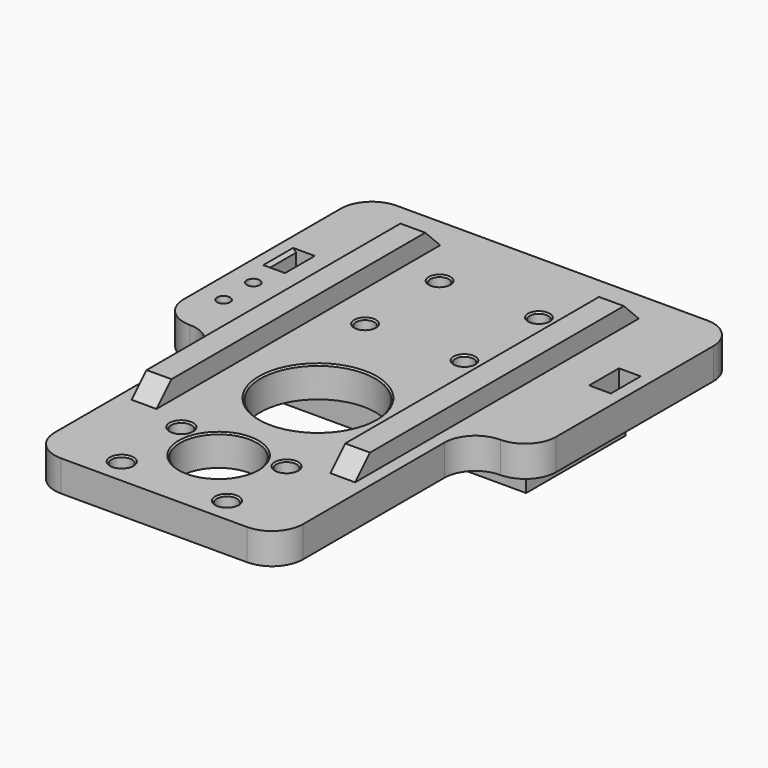
from build123d import *

# Parameters (mm, degrees)
F0_W         = 14.95
F0_H         = 5.5
F0_R         = 1.5
F0_H_2       = 4.5
F1_DEPTH     = 9.9
F3_R         = 1.65
F3_R_2       = 6.2
F3_R_3       = 9.25
F3_R_4       = 1.05
F3_R_5       = 1.5
F4_DEPTH     = 5
F5_SIZE2     = 0.25
F5_SIZE      = 0.25
F6_SIZE      = 0.5
F7_W         = 4
F7_H         = 61.1207796717
F8_DEPTH     = 3
F9_T4_DEPTH  = 29.7168298797
F9_T9_DEPTH  = 29.7168298797
F9_T14_DEPTH = 29.7168298797
F9_T19_DEPTH = 29.7168298797


# Not quite as in the source:
# - a fillet or chamfer that OpenCascade refuses, or shapes differently, is made with other operations: its cross-section is extruded or revolved along the edge and cut away or added


with BuildPart() as f1:
    # F0 (on Top) → F1 (new body)
    with BuildSketch(Plane.XY):
        with Locations((7.475, -7.25)):
            Rectangle(F0_W, F0_H)
        with Locations((8, -7.5)):
            Circle(F0_R, mode=Mode.SUBTRACT)
        with Locations((-7.475, -2.25)):
            Rectangle(F0_W, F0_H_2)
        Polygon((-19.95, 0), (-14.95, 0), (-14.95, 4.5), (-14.95, 10), (-19.95, 10), align=None)
        Polygon((-14.95, -4.5), (-14.95, 0), (-19.95, 0), (-19.95, -10), (-14.95, -10), align=None)
        Polygon((14.95, 4.5), (14.95, 0), (19.95, 0), (19.95, 10), (14.95, 10), align=None)
        Polygon((19.95, 0), (14.95, 0), (14.95, -4.5), (14.95, -10), (19.95, -10), align=None)
        with Locations((-7.475, -7.25)):
            Rectangle(F0_W, F0_H)
        with Locations((-8, -7.5)):
            Circle(F0_R, mode=Mode.SUBTRACT)
        with Locations((-7.475, 2.25)):
            Rectangle(F0_W, F0_H_2)
        with Locations((7.475, -2.25)):
            Rectangle(F0_W, F0_H_2)
        with Locations((7.475, 2.25)):
            Rectangle(F0_W, F0_H_2)
        with Locations((7.475, 7.25)):
            Rectangle(F0_W, F0_H)
        with Locations((8, 7.5)):
            Circle(F0_R, mode=Mode.SUBTRACT)
        with Locations((-7.475, 7.25)):
            Rectangle(F0_W, F0_H)
        with Locations((-8, 7.5)):
            Circle(F0_R, mode=Mode.SUBTRACT)
    extrude(amount=-F1_DEPTH)


with BuildPart() as f4:
    # F3 (on offset) → F4 (new body)
    with BuildSketch(Plane.XY.offset(-1)):
        with BuildLine():
            Line((25, 20.1207796717), (0, 20.1207796717))
            Line((0, 20.1207796717), (-25, 20.1207796717))
            ThreePointArc((-25, 20.1207796717), (-28.5355339059, 18.6563135776), (-30, 15.1207796717))
            Line((-30, 15.1207796717), (-30, -16.523957546))
            ThreePointArc((-30, -16.523957546), (-28.5355339059, -20.0594914519), (-25, -21.523957546))
            ThreePointArc((-25, -21.523957546), (-21.4644660941, -22.9884236401), (-20, -26.523957546))
            Line((-20, -26.523957546), (-20, -55))
            ThreePointArc((-20, -55), (-18.5355339059, -58.5355339059), (-15, -60))
            Line((-15, -60), (0, -60))
            Line((0, -60), (15, -60))
            ThreePointArc((15, -60), (18.5355339059, -58.5355339059), (20, -55))
            Line((20, -55), (20, -26.523957546))
            ThreePointArc((20, -26.523957546), (21.4644660941, -22.9884236401), (25, -21.523957546))
            ThreePointArc((25, -21.523957546), (28.5355339059, -20.0594914519), (30, -16.523957546))
            Line((30, -16.523957546), (30, 15.1207796717))
            ThreePointArc((30, 15.1207796717), (28.5355339059, 18.6563135776), (25, 20.1207796717))
        make_face()
        with Locations((-8.4598344365, -55.9289738999)):
            Circle(F3_R, mode=Mode.SUBTRACT)
        with Locations((-8.4598344365, -43.9289738999)):
            Circle(F3_R, mode=Mode.SUBTRACT)
        with Locations((8.5401655635, -55.9953450549)):
            Circle(F3_R, mode=Mode.SUBTRACT)
        with Locations((0, -47)):
            Circle(F3_R_2, mode=Mode.SUBTRACT)
        with Locations((8.5401655635, -43.9953450549)):
            Circle(F3_R, mode=Mode.SUBTRACT)
        with Locations((0, -27)):
            Circle(F3_R_3, mode=Mode.SUBTRACT)
        with Locations((-26, -13.5)):
            Circle(F3_R_4, mode=Mode.SUBTRACT)
        with Locations((-26, -7.5)):
            Circle(F3_R_4, mode=Mode.SUBTRACT)
        Polygon((-27.5, -3), (-27.5, 0), (-27.5, 3), (-24.5, 3), (-24.5, 0), (-24.5, -3), align=None, mode=Mode.SUBTRACT)
        with Locations((-8, -7.5)):
            Circle(F3_R_5, mode=Mode.SUBTRACT)
        with Locations((-8, 7.5)):
            Circle(F3_R_5, mode=Mode.SUBTRACT)
        with Locations((8, -7.5)):
            Circle(F3_R_5, mode=Mode.SUBTRACT)
        Polygon((24.5, 0), (24.5, 3), (27.5, 3), (27.5, 0), (27.5, -3), (24.5, -3), align=None, mode=Mode.SUBTRACT)
        with Locations((8, 7.5)):
            Circle(F3_R_5, mode=Mode.SUBTRACT)
    extrude(amount=F4_DEPTH)

    # F5
    f5_edges = [f4.edges().sort_by_distance(p)[0] for p in [
        (6.5, -7.5, 4),
        (6.5, 7.5, 4),
        (-9.5, 7.5, 4),
        (-9.5, -7.5, 4),
        (-10.109834, -43.928974, 4),
        (6.890166, -43.995345, 4),
        (6.890166, -55.995345, 4),
        (-10.109834, -55.928974, 4),
        (-6.2, -47, 4),
        (-9.25, -27, 4),
    ]]
    chamfer(f5_edges, length=F5_SIZE, length2=F5_SIZE2)

    # F6
    f6_edges = [f4.edges().sort_by_distance(p)[0] for p in [
        (-27.5, 0, 4),
        (27.5, 0, 4),
    ]]
    chamfer(f6_edges, length=F6_SIZE)

    # F7 (on face) → F8 (join)
    with BuildSketch(Plane.XY.offset(4)):
        with Locations((-16, -13.4396101642)):
            Rectangle(F7_W, F7_H)
        with Locations((16, -13.4396101642)):
            Rectangle(F7_W, F7_H)
    extrude(amount=F8_DEPTH)

    # F9: chamfer of 5 on 4 edges, made by hand


with BuildPart() as f9_tool2:
    # F9_s3 → F9_t4 (new body)
    with BuildSketch(Plane.YZ.offset(-30.8584149398)):
        Polygon((-39, 7), (-44, 2), (-44, 7), align=None)
    extrude(amount=F9_T4_DEPTH)

    split(bisect_by=Plane.XY.offset(4), keep=Keep.TOP)


with BuildPart() as f4_1:
    add(f4.part)

    # F9_t1: cut F9_tool2
    add(f9_tool2.part, mode=Mode.SUBTRACT)


with BuildPart() as f9_tool7:
    # F9_s8 → F9_t9 (new body)
    with BuildSketch(Plane.YZ.offset(1.1415850602)):
        Polygon((-39, 7), (-44, 2), (-44, 7), align=None)
    extrude(amount=F9_T9_DEPTH)

    split(bisect_by=Plane.XY.offset(4), keep=Keep.TOP)


with BuildPart() as f4_2:
    add(f4_1.part)

    # F9_t6: cut F9_tool7
    add(f9_tool7.part, mode=Mode.SUBTRACT)


with BuildPart() as f9_tool12:
    # F9_s13 → F9_t14 (new body)
    with BuildSketch(Plane.YZ.offset(-1.1415850602)):
        Polygon((12.1207796717, 7), (17.1207796717, 2), (17.1207796717, 7), align=None)
    extrude(amount=-F9_T14_DEPTH)

    split(bisect_by=Plane.XY.offset(4), keep=Keep.TOP)


with BuildPart() as f4_3:
    add(f4_2.part)

    # F9_t11: cut F9_tool12
    add(f9_tool12.part, mode=Mode.SUBTRACT)


with BuildPart() as f9_tool17:
    # F9_s18 → F9_t19 (new body)
    with BuildSketch(Plane.YZ.offset(30.8584149398)):
        Polygon((12.1207796717, 7), (17.1207796717, 2), (17.1207796717, 7), align=None)
    extrude(amount=-F9_T19_DEPTH)

    split(bisect_by=Plane.XY.offset(4), keep=Keep.TOP)


with BuildPart() as f4_4:
    add(f4_3.part)

    # F9_t16: cut F9_tool17
    add(f9_tool17.part, mode=Mode.SUBTRACT)


solid = Compound([f1.part, f4_4.part])
